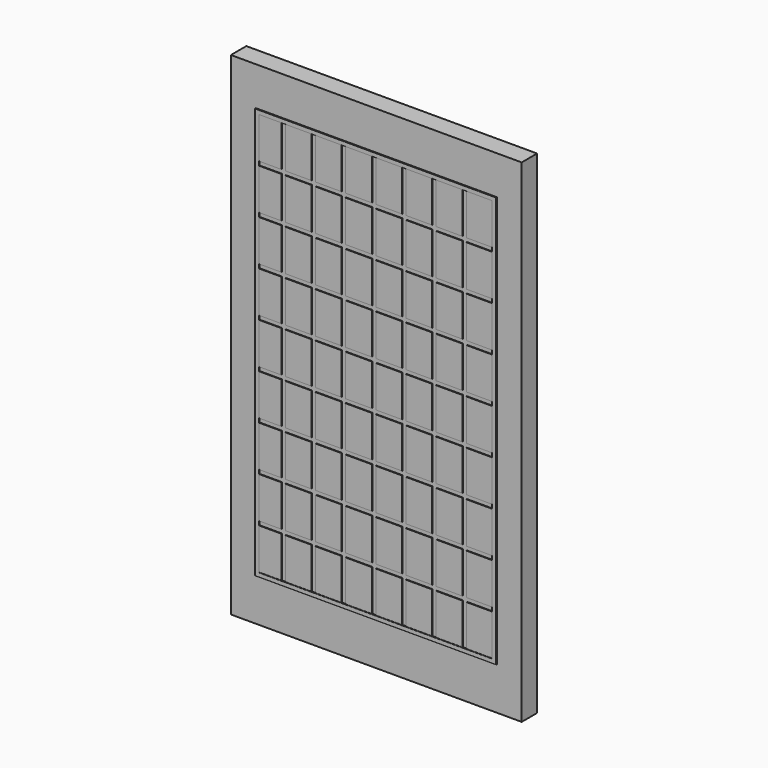
from build123d import *

# Parameters (mm, degrees)
F0_W     = 244.856
F0_H     = 414.782
F2_DEPTH = 16.256
F1_W     = 22.0209295034
F1_H     = 34.7209272623
F1_W_2   = 22.0208795034
F1_W_3   = 22.0208295034
F1_W_4   = 22.0207795034
F1_W_5   = 22.0207295034
F1_W_6   = 22.0206795034
F1_W_7   = 22.0206295034
F1_W_8   = 18.6415090069
F3_DEPTH = 16.764
F4_DEPTH = 17.018


# Not quite as in the source:
# - a pattern or mirror of a feature is missing from the dataset's text; its kind, count and spacing are read off the source's solid


with BuildPart() as f2:
    # F0 (on Front) → F2 (new body)
    with BuildSketch(Plane.XZ):
        Rectangle(F0_W, F0_H)
    extrude(amount=F2_DEPTH)

    # F1 (on face) → F3 (join)
    with BuildSketch(Plane.XZ):
        Polygon((76.2, -171.45), (101.6, -171.45), (101.6, -133.35), (101.6, -95.25), (101.6, -57.15), (101.6, -19.05), (101.6, 19.05), (101.6, 57.15), (101.6, 95.25), (101.6, 133.35), (101.6, 171.45), (101.6, 174.8282), (98.2209295034, 174.8282), (-101.6, 174.8282), (-101.6, 171.45), (-101.6, 133.35), (-101.6, -171.45), (-76.2, -171.45), (-50.8, -171.45), (-25.4, -171.45), (0, -171.45), (25.4, -171.45), (50.8, -171.45), align=None)
        Polygon((76.2, 171.45), (98.2209295034, 171.45), (98.2209295034, 136.7290727377), (98.2209295034, 133.35), (98.2209295034, 98.6290727377), (98.2209295034, 95.25), (98.2209295034, 60.5290727377), (98.2209295034, 57.15), (98.2209295034, 22.4290727377), (98.2209295034, 19.05), (98.2209295034, -15.6709272623), (98.2209295034, -19.05), (98.2209295034, -53.7709272623), (98.2209295034, -57.15), (98.2209295034, -91.8709272623), (98.2209295034, -95.25), (98.2209295034, -129.9709272623), (98.2209295034, -133.35), (98.2209295034, -168.0709272623), (76.2, -168.0709272623), (72.8208795034, -168.0709272623), (50.8, -168.0709272623), (47.4208295034, -168.0709272623), (25.4, -168.0709272623), (22.0207795034, -168.0709272623), (0, -168.0709272623), (-3.3792704966, -168.0709272623), (-25.4, -168.0709272623), (-28.7793204966, -168.0709272623), (-50.8, -168.0709272623), (-54.1793704966, -168.0709272623), (-76.2, -168.0709272623), (-79.5794204966, -168.0709272623), (-98.2209295034, -168.0709272623), (-98.2209295034, -133.35), (-98.2209295034, -129.9709272623), (-98.2209295034, -95.25), (-98.2209295034, -91.8709272623), (-98.2209295034, -57.15), (-98.2209295034, -53.7709272623), (-98.2209295034, -19.05), (-98.2209295034, -15.6709272623), (-98.2209295034, 19.05), (-98.2209295034, 22.4290727377), (-98.2209295034, 57.15), (-98.2209295034, 60.5290727377), (-98.2209295034, 95.25), (-98.2209295034, 98.6290727377), (-98.2209295034, 133.35), (-98.2209295034, 136.7290727377), (-98.2209295034, 171.45), (-79.5794204966, 171.45), (-76.2, 171.45), (-54.1793704966, 171.45), (-50.8, 171.45), (-28.7793204966, 171.45), (-25.4, 171.45), (-3.3792704966, 171.45), (0, 171.45), (22.0207795034, 171.45), (25.4, 171.45), (47.4208295034, 171.45), (50.8, 171.45), (72.8208795034, 171.45), align=None, mode=Mode.SUBTRACT)
        with Locations((87.2104647517, 154.0895363688)):
            Rectangle(F1_W, F1_H)
        with Locations((87.2104647517, 115.9895363688)):
            Rectangle(F1_W, F1_H)
        with Locations((87.2104647517, 77.8895363688)):
            Rectangle(F1_W, F1_H)
        with Locations((87.2104647517, 39.7895363688)):
            Rectangle(F1_W, F1_H)
        with Locations((87.2104647517, 1.6895363688)):
            Rectangle(F1_W, F1_H)
        with Locations((87.2104647517, -36.4104636312)):
            Rectangle(F1_W, F1_H)
        with Locations((87.2104647517, -74.5104636312)):
            Rectangle(F1_W, F1_H)
        with Locations((87.2104647517, -112.6104636312)):
            Rectangle(F1_W, F1_H)
        with Locations((87.2104647517, -150.7104636312)):
            Rectangle(F1_W, F1_H)
        with Locations((61.8104397517, -150.7104636312)):
            Rectangle(F1_W_2, F1_H)
        with Locations((61.8104397517, -112.6104636312)):
            Rectangle(F1_W_2, F1_H)
        with Locations((61.8104397517, -74.5104636312)):
            Rectangle(F1_W_2, F1_H)
        with Locations((61.8104397517, -36.4104636312)):
            Rectangle(F1_W_2, F1_H)
        with Locations((61.8104397517, 1.6895363688)):
            Rectangle(F1_W_2, F1_H)
        with Locations((61.8104397517, 39.7895363688)):
            Rectangle(F1_W_2, F1_H)
        with Locations((61.8104397517, 77.8895363688)):
            Rectangle(F1_W_2, F1_H)
        with Locations((61.8104397517, 115.9895363688)):
            Rectangle(F1_W_2, F1_H)
        with Locations((61.8104397517, 154.0895363688)):
            Rectangle(F1_W_2, F1_H)
        with Locations((36.4104147517, 154.0895363688)):
            Rectangle(F1_W_3, F1_H)
        with Locations((36.4104147517, 115.9895363688)):
            Rectangle(F1_W_3, F1_H)
        with Locations((36.4104147517, 77.8895363688)):
            Rectangle(F1_W_3, F1_H)
        with Locations((36.4104147517, 39.7895363688)):
            Rectangle(F1_W_3, F1_H)
        with Locations((36.4104147517, 1.6895363688)):
            Rectangle(F1_W_3, F1_H)
        with Locations((36.4104147517, -36.4104636312)):
            Rectangle(F1_W_3, F1_H)
        with Locations((36.4104147517, -74.5104636312)):
            Rectangle(F1_W_3, F1_H)
        with Locations((36.4104147517, -112.6104636312)):
            Rectangle(F1_W_3, F1_H)
        with Locations((36.4104147517, -150.7104636312)):
            Rectangle(F1_W_3, F1_H)
        with Locations((11.0103897517, 154.0895363688)):
            Rectangle(F1_W_4, F1_H)
        with Locations((11.0103897517, 115.9895363688)):
            Rectangle(F1_W_4, F1_H)
        with Locations((11.0103897517, 77.8895363688)):
            Rectangle(F1_W_4, F1_H)
        with Locations((11.0103897517, 39.7895363688)):
            Rectangle(F1_W_4, F1_H)
        with Locations((11.0103897517, 1.6895363688)):
            Rectangle(F1_W_4, F1_H)
        with Locations((11.0103897517, -36.4104636312)):
            Rectangle(F1_W_4, F1_H)
        with Locations((11.0103897517, -74.5104636312)):
            Rectangle(F1_W_4, F1_H)
        with Locations((11.0103897517, -112.6104636312)):
            Rectangle(F1_W_4, F1_H)
        with Locations((11.0103897517, -150.7104636312)):
            Rectangle(F1_W_4, F1_H)
        with Locations((-14.3896352483, 154.0895363688)):
            Rectangle(F1_W_5, F1_H)
        with Locations((-14.3896352483, 115.9895363688)):
            Rectangle(F1_W_5, F1_H)
        with Locations((-14.3896352483, 77.8895363688)):
            Rectangle(F1_W_5, F1_H)
        with Locations((-14.3896352483, 39.7895363688)):
            Rectangle(F1_W_5, F1_H)
        with Locations((-14.3896352483, 1.6895363688)):
            Rectangle(F1_W_5, F1_H)
        with Locations((-14.3896352483, -36.4104636312)):
            Rectangle(F1_W_5, F1_H)
        with Locations((-14.3896352483, -74.5104636312)):
            Rectangle(F1_W_5, F1_H)
        with Locations((-14.3896352483, -112.6104636312)):
            Rectangle(F1_W_5, F1_H)
        with Locations((-14.3896352483, -150.7104636312)):
            Rectangle(F1_W_5, F1_H)
        with Locations((-39.7896602483, 154.0895363688)):
            Rectangle(F1_W_6, F1_H)
        with Locations((-39.7896602483, 115.9895363688)):
            Rectangle(F1_W_6, F1_H)
        with Locations((-39.7896602483, 77.8895363688)):
            Rectangle(F1_W_6, F1_H)
        with Locations((-39.7896602483, 39.7895363688)):
            Rectangle(F1_W_6, F1_H)
        with Locations((-39.7896602483, 1.6895363688)):
            Rectangle(F1_W_6, F1_H)
        with Locations((-39.7896602483, -36.4104636312)):
            Rectangle(F1_W_6, F1_H)
        with Locations((-39.7896602483, -74.5104636312)):
            Rectangle(F1_W_6, F1_H)
        with Locations((-39.7896602483, -112.6104636312)):
            Rectangle(F1_W_6, F1_H)
        with Locations((-39.7896602483, -150.7104636312)):
            Rectangle(F1_W_6, F1_H)
        with Locations((-65.1896852483, 154.0895363688)):
            Rectangle(F1_W_7, F1_H)
        with Locations((-65.1896852483, 115.9895363688)):
            Rectangle(F1_W_7, F1_H)
        with Locations((-65.1896852483, 77.8895363688)):
            Rectangle(F1_W_7, F1_H)
        with Locations((-65.1896852483, 39.7895363688)):
            Rectangle(F1_W_7, F1_H)
        with Locations((-65.1896852483, 1.6895363688)):
            Rectangle(F1_W_7, F1_H)
        with Locations((-65.1896852483, -36.4104636312)):
            Rectangle(F1_W_7, F1_H)
        with Locations((-65.1896852483, -74.5104636312)):
            Rectangle(F1_W_7, F1_H)
        with Locations((-65.1896852483, -112.6104636312)):
            Rectangle(F1_W_7, F1_H)
        with Locations((-65.1896852483, -150.7104636312)):
            Rectangle(F1_W_7, F1_H)
        with Locations((-88.900175, 115.9895363688)):
            Rectangle(F1_W_8, F1_H)
        with Locations((-88.900175, 77.8895363688)):
            Rectangle(F1_W_8, F1_H)
        with Locations((-88.900175, 39.7895363688)):
            Rectangle(F1_W_8, F1_H)
        with Locations((-88.900175, 1.6895363688)):
            Rectangle(F1_W_8, F1_H)
        with Locations((-88.900175, -36.4104636312)):
            Rectangle(F1_W_8, F1_H)
        with Locations((-88.900175, -74.5104636312)):
            Rectangle(F1_W_8, F1_H)
        with Locations((-88.900175, -112.6104636312)):
            Rectangle(F1_W_8, F1_H)
        with Locations((-88.900175, -150.7104636312)):
            Rectangle(F1_W_8, F1_H)
    f3 = extrude(amount=F3_DEPTH)

    # F3_copies: F3 across plane
    add(f3.mirror(Plane.XY.offset(1.689536)))

    # F1 (on face) → F4 (join)
    with BuildSketch(Plane.XZ):
        Polygon((76.2, -171.45), (101.6, -171.45), (101.6, -133.35), (101.6, -95.25), (101.6, -57.15), (101.6, -19.05), (101.6, 19.05), (101.6, 57.15), (101.6, 95.25), (101.6, 133.35), (101.6, 171.45), (101.6, 174.8282), (98.2209295034, 174.8282), (-101.6, 174.8282), (-101.6, 171.45), (-101.6, 133.35), (-101.6, -171.45), (-76.2, -171.45), (-50.8, -171.45), (-25.4, -171.45), (0, -171.45), (25.4, -171.45), (50.8, -171.45), align=None)
        Polygon((76.2, 171.45), (98.2209295034, 171.45), (98.2209295034, 136.7290727377), (98.2209295034, 133.35), (98.2209295034, 98.6290727377), (98.2209295034, 95.25), (98.2209295034, 60.5290727377), (98.2209295034, 57.15), (98.2209295034, 22.4290727377), (98.2209295034, 19.05), (98.2209295034, -15.6709272623), (98.2209295034, -19.05), (98.2209295034, -53.7709272623), (98.2209295034, -57.15), (98.2209295034, -91.8709272623), (98.2209295034, -95.25), (98.2209295034, -129.9709272623), (98.2209295034, -133.35), (98.2209295034, -168.0709272623), (76.2, -168.0709272623), (72.8208795034, -168.0709272623), (50.8, -168.0709272623), (47.4208295034, -168.0709272623), (25.4, -168.0709272623), (22.0207795034, -168.0709272623), (0, -168.0709272623), (-3.3792704966, -168.0709272623), (-25.4, -168.0709272623), (-28.7793204966, -168.0709272623), (-50.8, -168.0709272623), (-54.1793704966, -168.0709272623), (-76.2, -168.0709272623), (-79.5794204966, -168.0709272623), (-98.2209295034, -168.0709272623), (-98.2209295034, -133.35), (-98.2209295034, -129.9709272623), (-98.2209295034, -95.25), (-98.2209295034, -91.8709272623), (-98.2209295034, -57.15), (-98.2209295034, -53.7709272623), (-98.2209295034, -19.05), (-98.2209295034, -15.6709272623), (-98.2209295034, 19.05), (-98.2209295034, 22.4290727377), (-98.2209295034, 57.15), (-98.2209295034, 60.5290727377), (-98.2209295034, 95.25), (-98.2209295034, 98.6290727377), (-98.2209295034, 133.35), (-98.2209295034, 136.7290727377), (-98.2209295034, 171.45), (-79.5794204966, 171.45), (-76.2, 171.45), (-54.1793704966, 171.45), (-50.8, 171.45), (-28.7793204966, 171.45), (-25.4, 171.45), (-3.3792704966, 171.45), (0, 171.45), (22.0207795034, 171.45), (25.4, 171.45), (47.4208295034, 171.45), (50.8, 171.45), (72.8208795034, 171.45), align=None, mode=Mode.SUBTRACT)
    extrude(amount=F4_DEPTH)


solid = f2.part
